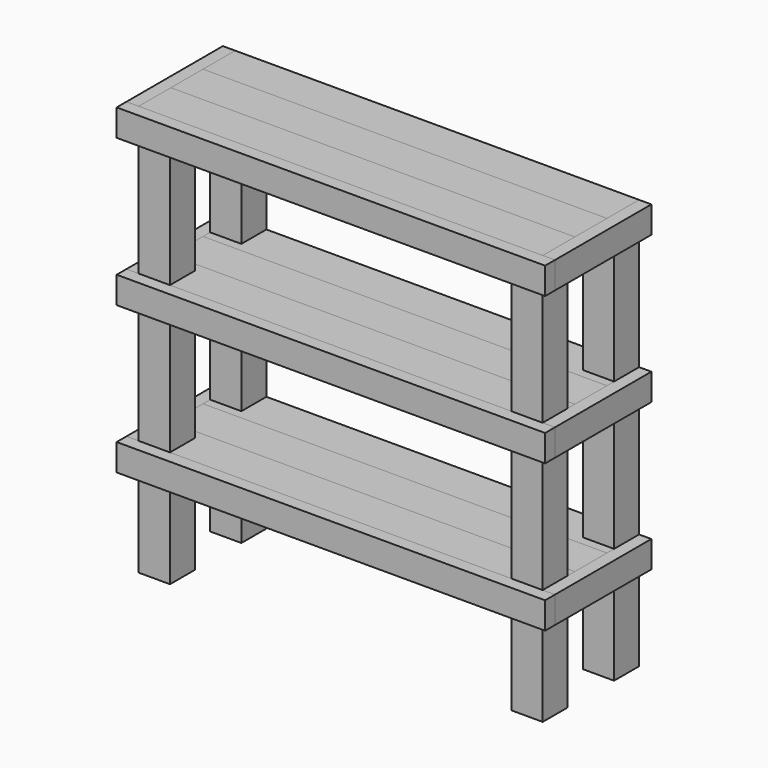
from build123d import *

# Parameters (mm, degrees)
F0_W      = 88.9
F0_H      = 88.9
F1_DEPTH  = 1168.4
F2_W      = 25.4
F2_H      = 38.1
F2_W_2    = 88.9
F3_DEPTH  = 1149.35
F2_W_3    = 114.3
F4_DEPTH  = 1149.35
F5_W      = 63.5
F5_H      = 63.5
F6_DEPTH  = 1168.401
F8_W      = 34.925
F8_H      = 76.2
F9_DEPTH  = 342.9
F10_W     = 1219.2
F10_H     = 76.2
F11_DEPTH = 34.925


with BuildPart() as f1:
    # F0 (on Top) → F1 (new body)
    with BuildSketch(Plane.XY):
        with Locations((44.45, 44.45)):
            Rectangle(F0_W, F0_H)
    extrude(amount=F1_DEPTH)


with BuildPart() as f1b:
    # F0 (on Top) → F1, piece 2 (new body)
    with BuildSketch(Plane.XY):
        with Locations((1104.9, 44.45)):
            Rectangle(F0_W, F0_H)
    extrude(amount=F1_DEPTH)


with BuildPart() as f1c:
    # F0 (on Top) → F1, piece 3 (new body)
    with BuildSketch(Plane.XY):
        with Locations((44.45, 298.45)):
            Rectangle(F0_W, F0_H)
    extrude(amount=F1_DEPTH)


with BuildPart() as f1d:
    # F0 (on Top) → F1, piece 4 (new body)
    with BuildSketch(Plane.XY):
        with Locations((1104.9, 298.45)):
            Rectangle(F0_W, F0_H)
    extrude(amount=F1_DEPTH)


with BuildPart() as f3:
    # F2 (on face) → F3 (new body, through all)
    with BuildSketch(Plane(origin=(0, 0, 0), x_dir=(0, -1, 0), z_dir=(-1, 0, 0))):
        with Locations((-241.3, 1149.35)):
            Rectangle(F2_W, F2_H)
        with Locations((-298.45, 1149.35)):
            Rectangle(F2_W_2, F2_H)
    extrude(amount=-F3_DEPTH)


with BuildPart() as f3b:
    # F2 (on face) → F3, piece 2 (new body, through all)
    with BuildSketch(Plane(origin=(0, 0, 0), x_dir=(0, -1, 0), z_dir=(-1, 0, 0))):
        with Locations((-57.15, 1149.35)):
            Rectangle(F2_W_3, F2_H)
    extrude(amount=-F3_DEPTH)


with BuildPart() as f3c:
    # F2 (on face) → F3, piece 3 (new body, through all)
    with BuildSketch(Plane(origin=(0, 0, 0), x_dir=(0, -1, 0), z_dir=(-1, 0, 0))):
        with Locations((-298.45, 730.25)):
            Rectangle(F2_W_2, F2_H)
        with Locations((-241.3, 730.25)):
            Rectangle(F2_W, F2_H)
    extrude(amount=-F3_DEPTH)


with BuildPart() as f3d:
    # F2 (on face) → F3, piece 4 (new body, through all)
    with BuildSketch(Plane(origin=(0, 0, 0), x_dir=(0, -1, 0), z_dir=(-1, 0, 0))):
        with Locations((-298.45, 311.15)):
            Rectangle(F2_W_2, F2_H)
        with Locations((-241.3, 311.15)):
            Rectangle(F2_W, F2_H)
    extrude(amount=-F3_DEPTH)


with BuildPart() as f3e:
    # F2 (on face) → F3, piece 5 (new body, through all)
    with BuildSketch(Plane(origin=(0, 0, 0), x_dir=(0, -1, 0), z_dir=(-1, 0, 0))):
        with Locations((-57.15, 311.15)):
            Rectangle(F2_W_3, F2_H)
    extrude(amount=-F3_DEPTH)


with BuildPart() as f3f:
    # F2 (on face) → F3, piece 6 (new body, through all)
    with BuildSketch(Plane(origin=(0, 0, 0), x_dir=(0, -1, 0), z_dir=(-1, 0, 0))):
        with Locations((-57.15, 730.25)):
            Rectangle(F2_W_3, F2_H)
    extrude(amount=-F3_DEPTH)


with BuildPart() as f4:
    # F2 (on face) → F4 (new body, through all)
    with BuildSketch(Plane(origin=(0, 0, 0), x_dir=(0, -1, 0), z_dir=(-1, 0, 0))):
        with Locations((-171.45, 1149.35)):
            Rectangle(F2_W_3, F2_H)
    extrude(amount=-F4_DEPTH)


with BuildPart() as f4b:
    # F2 (on face) → F4, piece 2 (new body, through all)
    with BuildSketch(Plane(origin=(0, 0, 0), x_dir=(0, -1, 0), z_dir=(-1, 0, 0))):
        with Locations((-171.45, 730.25)):
            Rectangle(F2_W_3, F2_H)
    extrude(amount=-F4_DEPTH)


with BuildPart() as f4c:
    # F2 (on face) → F4, piece 3 (new body, through all)
    with BuildSketch(Plane(origin=(0, 0, 0), x_dir=(0, -1, 0), z_dir=(-1, 0, 0))):
        with Locations((-171.45, 311.15)):
            Rectangle(F2_W_3, F2_H)
    extrude(amount=-F4_DEPTH)


with BuildPart() as f6_tool:
    # F5 (on face) → F6 (new body, through all)
    with BuildSketch(Plane.XY.offset(1168.4)):
        with Locations((31.75, 31.75)):
            Rectangle(F5_W, F5_H)
        with Locations((1117.6, 31.75)):
            Rectangle(F5_W, F5_H)
        with Locations((1117.6, 311.15)):
            Rectangle(F5_W, F5_H)
        with Locations((31.75, 311.15)):
            Rectangle(F5_W, F5_H)
    extrude(amount=-F6_DEPTH)


with BuildPart() as f3c_1:
    add(f3c.part)

    # F6: cut by f6_tool
    add(f6_tool.part, mode=Mode.SUBTRACT)


with BuildPart() as f3d_1:
    add(f3d.part)

    # F6: cut by f6_tool
    add(f6_tool.part, mode=Mode.SUBTRACT)


with BuildPart() as f3e_1:
    add(f3e.part)

    # F6: cut by f6_tool
    add(f6_tool.part, mode=Mode.SUBTRACT)


with BuildPart() as f3f_1:
    add(f3f.part)

    # F6: cut by f6_tool
    add(f6_tool.part, mode=Mode.SUBTRACT)


with BuildPart() as f1c_1:
    add(f1c.part)

    # F7: cut F3c, F3f, F3d, F3e, F3, F3b
    add(f3c_1.part, mode=Mode.SUBTRACT)
    add(f3f_1.part, mode=Mode.SUBTRACT)
    add(f3d_1.part, mode=Mode.SUBTRACT)
    add(f3e_1.part, mode=Mode.SUBTRACT)
    add(f3.part, mode=Mode.SUBTRACT)
    add(f3b.part, mode=Mode.SUBTRACT)


with BuildPart() as f1_1:
    add(f1.part)

    # F7: cut F3c, F3f, F3d, F3e, F3, F3b
    add(f3c_1.part, mode=Mode.SUBTRACT)
    add(f3f_1.part, mode=Mode.SUBTRACT)
    add(f3d_1.part, mode=Mode.SUBTRACT)
    add(f3e_1.part, mode=Mode.SUBTRACT)
    add(f3.part, mode=Mode.SUBTRACT)
    add(f3b.part, mode=Mode.SUBTRACT)


with BuildPart() as f1d_1:
    add(f1d.part)

    # F7: cut F3c, F3f, F3d, F3e, F3, F3b
    add(f3c_1.part, mode=Mode.SUBTRACT)
    add(f3f_1.part, mode=Mode.SUBTRACT)
    add(f3d_1.part, mode=Mode.SUBTRACT)
    add(f3e_1.part, mode=Mode.SUBTRACT)
    add(f3.part, mode=Mode.SUBTRACT)
    add(f3b.part, mode=Mode.SUBTRACT)


with BuildPart() as f1b_1:
    add(f1b.part)

    # F7: cut F3c, F3f, F3d, F3e, F3, F3b
    add(f3c_1.part, mode=Mode.SUBTRACT)
    add(f3f_1.part, mode=Mode.SUBTRACT)
    add(f3d_1.part, mode=Mode.SUBTRACT)
    add(f3e_1.part, mode=Mode.SUBTRACT)
    add(f3.part, mode=Mode.SUBTRACT)
    add(f3b.part, mode=Mode.SUBTRACT)


with BuildPart() as f9:
    # F8 (on face) → F9 (new body, through all)
    with BuildSketch(Plane(origin=(0, 342.9, 0), x_dir=(-1, 0, 0), z_dir=(0, 1, 0))):
        with Locations((-1166.8125, 1130.3)):
            Rectangle(F8_W, F8_H)
    extrude(amount=-F9_DEPTH)


with BuildPart() as f9b:
    # F8 (on face) → F9, piece 2 (new body, through all)
    with BuildSketch(Plane(origin=(0, 342.9, 0), x_dir=(-1, 0, 0), z_dir=(0, 1, 0))):
        with Locations((-1166.8125, 711.2)):
            Rectangle(F8_W, F8_H)
    extrude(amount=-F9_DEPTH)


with BuildPart() as f9c:
    # F8 (on face) → F9, piece 3 (new body, through all)
    with BuildSketch(Plane(origin=(0, 342.9, 0), x_dir=(-1, 0, 0), z_dir=(0, 1, 0))):
        with Locations((-1166.8125, 292.1)):
            Rectangle(F8_W, F8_H)
    extrude(amount=-F9_DEPTH)


with BuildPart() as f9d:
    # F8 (on face) → F9, piece 4 (new body, through all)
    with BuildSketch(Plane(origin=(0, 342.9, 0), x_dir=(-1, 0, 0), z_dir=(0, 1, 0))):
        with Locations((17.4625, 1130.3)):
            Rectangle(F8_W, F8_H)
    extrude(amount=-F9_DEPTH)


with BuildPart() as f9e:
    # F8 (on face) → F9, piece 5 (new body, through all)
    with BuildSketch(Plane(origin=(0, 342.9, 0), x_dir=(-1, 0, 0), z_dir=(0, 1, 0))):
        with Locations((17.4625, 711.2)):
            Rectangle(F8_W, F8_H)
    extrude(amount=-F9_DEPTH)


with BuildPart() as f9f:
    # F8 (on face) → F9, piece 6 (new body, through all)
    with BuildSketch(Plane(origin=(0, 342.9, 0), x_dir=(-1, 0, 0), z_dir=(0, 1, 0))):
        with Locations((17.4625, 292.1)):
            Rectangle(F8_W, F8_H)
    extrude(amount=-F9_DEPTH)


with BuildPart() as f11:
    # F10 (on face) → F11 (new body)
    with BuildSketch(Plane.XZ):
        with Locations((574.675, 292.1)):
            Rectangle(F10_W, F10_H)
    extrude(amount=F11_DEPTH)


with BuildPart() as f11b:
    # F10 (on face) → F11, piece 2 (new body)
    with BuildSketch(Plane.XZ):
        with Locations((574.675, 711.2)):
            Rectangle(F10_W, F10_H)
    extrude(amount=F11_DEPTH)


with BuildPart() as f11c:
    # F10 (on face) → F11, piece 3 (new body)
    with BuildSketch(Plane.XZ):
        with Locations((574.675, 1130.3)):
            Rectangle(F10_W, F10_H)
    extrude(amount=F11_DEPTH)


solid = Compound([f3.part, f3b.part, f4.part, f4b.part, f4c.part, f3c_1.part, f3d_1.part, f3e_1.part, f3f_1.part, f1c_1.part, f1_1.part, f1d_1.part, f1b_1.part, f9.part, f9b.part, f9c.part, f9d.part, f9e.part, f9f.part, f11.part, f11b.part, f11c.part])
